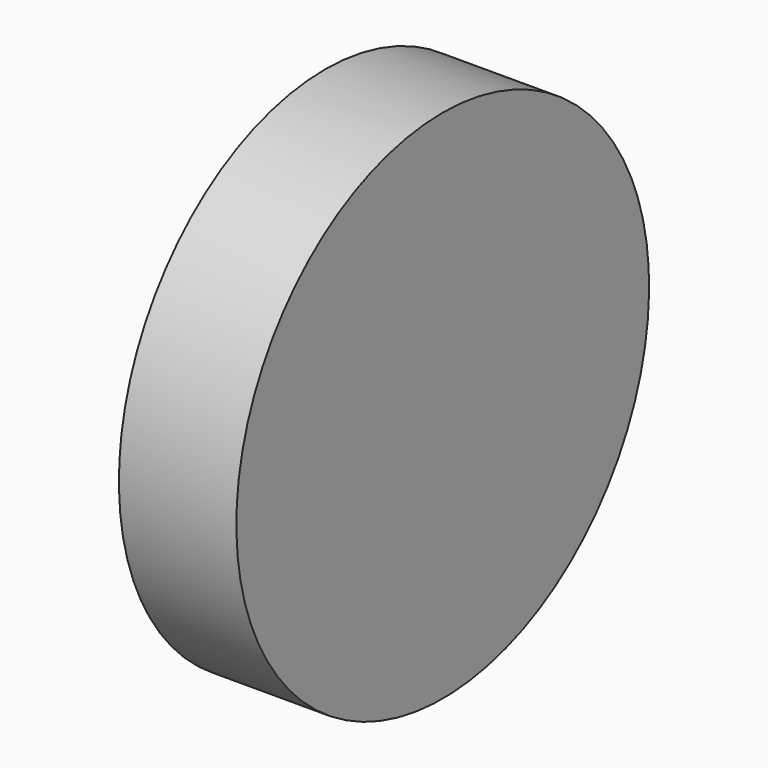
from build123d import *


with BuildPart() as f1:
    # F0 (on Front) → F1 (revolve)
    with BuildSketch(Plane.XZ):
        with BuildLine():
            add(Edge.make_bspline(
                [(-10.9723351412, 26.4565628022), (-10.3018910534, 26.4624551956), (-9.4257966097, 26.0553417029), (-8.2234851438, 25.1009661647), (-8.0662317018, 24.8820760133), (-7.9947902337, 24.7891377658)],
                knots=[0.3661893236, 0.3661893236, 0.3661893236, 0.3661893236, 0.63187276, 0.8763069792, 1, 1, 1, 1], degree=3))
            Line((-7.9947902337, 24.7891377658), (0, 15.100086289))
            Line((0, 15.100086289), (0, 0))
            Line((0, 0), (2, 0))
            Line((2, 0), (2, 28.4919212472))
            Line((2, 28.4919212472), (0, 28.4919212472))
            Line((0, 28.4919212472), (-10.9723351412, 28.4919212472))
            Line((-10.9723351412, 28.4919212472), (-10.9723351412, 26.4565628022))
        make_face()
    revolve(axis=Axis((1, 0, 0), (-1, 0, 0)))


solid = f1.part
